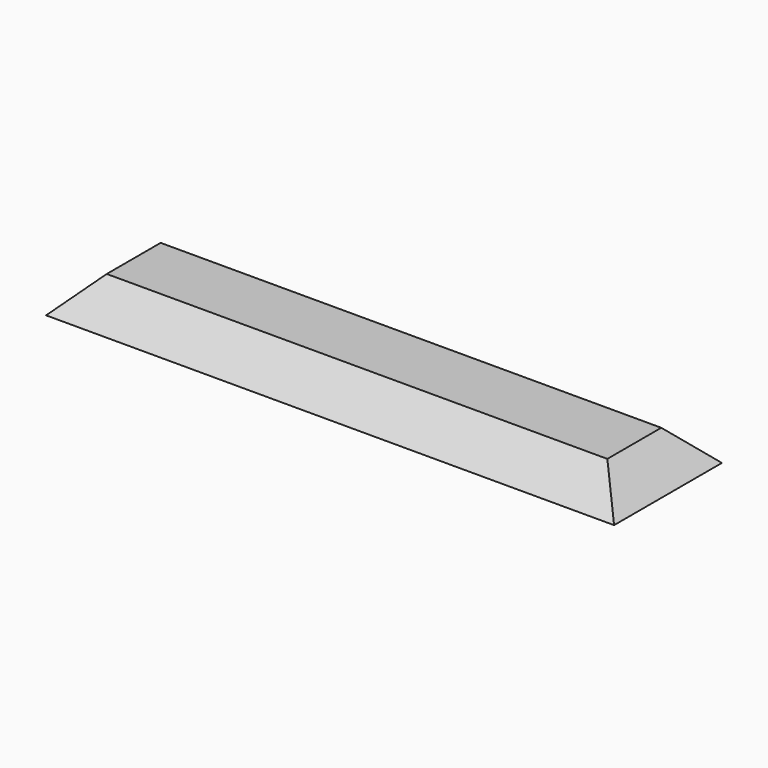
from build123d import *

# Parameters (mm, degrees)
F0_W        = 76.2
F0_H        = 19.05
F1_DEPTH    = 4.445
F3_T1_DEPTH = 102.3282991577
F3_T3_DEPTH = 45.1782991577


# Not quite as in the source:
# - a fillet or chamfer that OpenCascade refuses, or shapes differently, is made with other operations: its cross-section is extruded or revolved along the edge and cut away or added
# - a feature names something its author has since deleted; it is built from what else it names


with BuildPart() as f1:
    # F0 (on Top) → F1 (new body)
    with BuildSketch(Plane.XY):
        Rectangle(F0_W, F0_H)
    extrude(amount=F1_DEPTH)

    # F3: chamfer of 5.08 on 4 edges, made by hand

    # F3_s2 → F3_t1 (cut)
    with BuildSketch(Plane.YZ.offset(-51.1641495789)):
        Polygon((-9.525, -0.635), (-4.445, 4.445), (-9.525, 4.445), align=None)
        Polygon((9.525, -0.635), (4.445, 4.445), (9.525, 4.445), align=None)
    extrude(amount=F3_T1_DEPTH, mode=Mode.SUBTRACT)

    # F3_s4 → F3_t3 (cut)
    with BuildSketch(Plane.XZ.offset(-22.5891495789)):
        Polygon((-38.1, -0.635), (-33.02, 4.445), (-38.1, 4.445), align=None)
        Polygon((38.1, -0.635), (33.02, 4.445), (38.1, 4.445), align=None)
    extrude(amount=F3_T3_DEPTH, mode=Mode.SUBTRACT)


solid = f1.part
